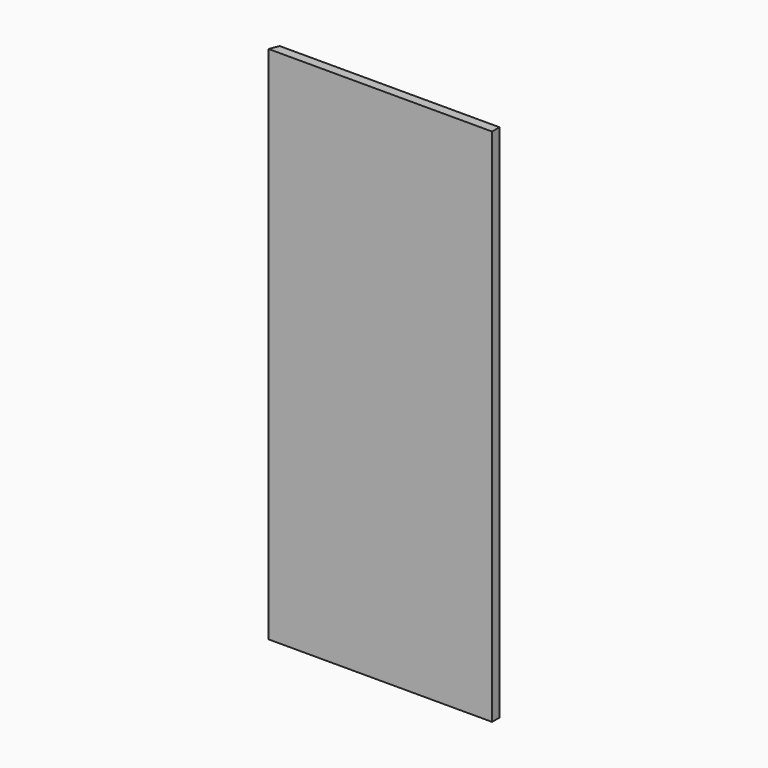
from build123d import *

# Parameters (mm, degrees)
F0_W     = 381
F0_H     = 885.825
F1_DEPTH = 15.875
F2_SIZE2 = 6.57563
F2_SIZE  = 15.87499


# Not quite as in the source:
# - a fillet or chamfer is up to 0.001 mm smaller than in the source, because OpenCascade refuses the exact size


with BuildPart() as f1:
    # F0 (on Front) → F1 (new body)
    with BuildSketch(Plane.XZ):
        with Locations((190.5, 442.9125)):
            Rectangle(F0_W, F0_H)
    extrude(amount=-F1_DEPTH)

    # F2 (size 15.875 and 6.5756403027 in the source; OpenCascade refuses exactly that, so slightly less here)
    f2_edges = [f1.edges().sort_by_distance(p)[0] for p in [
        (0, 15.875, 442.9125),
    ]]
    f2_side = f1.faces().sort_by_distance((0, 7.9375, 442.9125))[0]
    chamfer(f2_edges, length=F2_SIZE, length2=F2_SIZE2, reference=f2_side)


solid = f1.part
